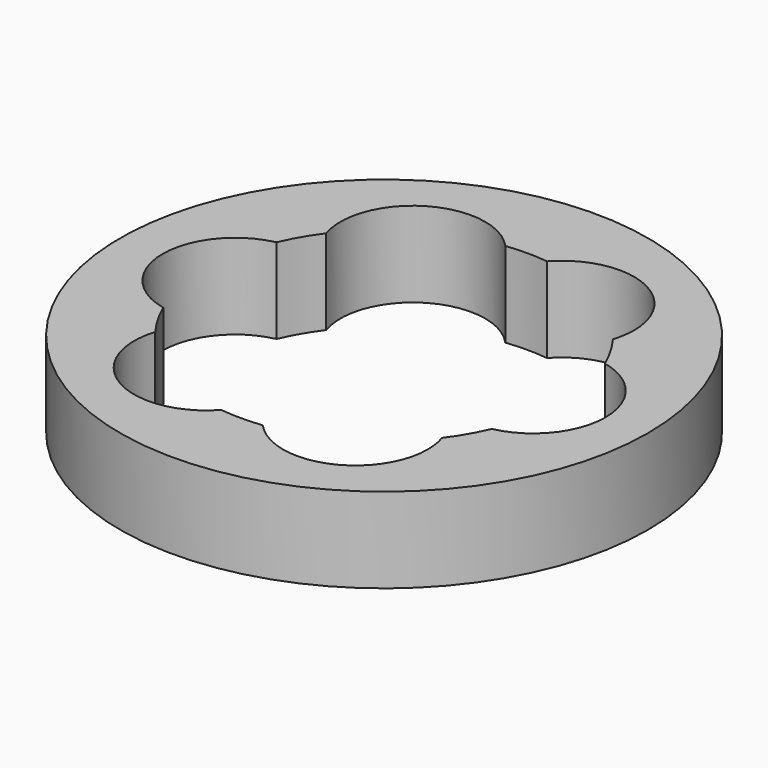
from build123d import *

# Parameters (mm, degrees)
F0_R     = 31
F1_DEPTH = 10


# Not quite as in the source:
# - a feature names something its author has since deleted; it is built from what else it names


with BuildPart() as f1:
    # F0 (on Top) → F1 (new body)
    with BuildSketch(Plane.XY):
        Circle(F0_R)
        with BuildLine():
            ThreePointArc((19.2857142857, 8.310308327), (24.1116779802, 5.3418830281), (26, 0))
            ThreePointArc((26, 0), (24.1116779802, -5.3418830281), (19.2857142857, -8.310308327))
            ThreePointArc((19.2857142857, -8.310308327), (18.1865334795, -10.5), (16.8397952673, -12.5467643381))
            ThreePointArc((16.8397952673, -12.5467643381), (17.1468226066, -13.83507715), (17.25, -15.1554445662))
            ThreePointArc((17.25, -15.1554445662), (11.8049395785, -23.0874899627), (2.4459190184, -20.8570726651))
            ThreePointArc((2.4459190184, -20.8570726651), (0, -21), (-2.4459190184, -20.8570726651))
            ThreePointArc((-2.4459190184, -20.8570726651), (-13, -22.5166604984), (-16.8397952673, -12.5467643381))
            ThreePointArc((-16.8397952673, -12.5467643381), (-18.1865334795, -10.5), (-19.2857142857, -8.310308327))
            ThreePointArc((-19.2857142857, -8.310308327), (-26, 0), (-19.2857142857, 8.310308327))
            ThreePointArc((-19.2857142857, 8.310308327), (-18.1865334795, 10.5), (-16.8397952673, 12.5467643381))
            ThreePointArc((-16.8397952673, 12.5467643381), (-13, 22.5166604984), (-2.4459190184, 20.8570726651))
            ThreePointArc((-2.4459190184, 20.8570726651), (0, 21), (2.4459190184, 20.8570726651))
            ThreePointArc((2.4459190184, 20.8570726651), (11.8049395785, 23.0874899627), (17.25, 15.1554445662))
            ThreePointArc((17.25, 15.1554445662), (17.1468226066, 13.83507715), (16.8397952673, 12.5467643381))
            ThreePointArc((16.8397952673, 12.5467643381), (18.1865334795, 10.5), (19.2857142857, 8.310308327))
        make_face(mode=Mode.SUBTRACT)
    extrude(amount=F1_DEPTH)


solid = f1.part
